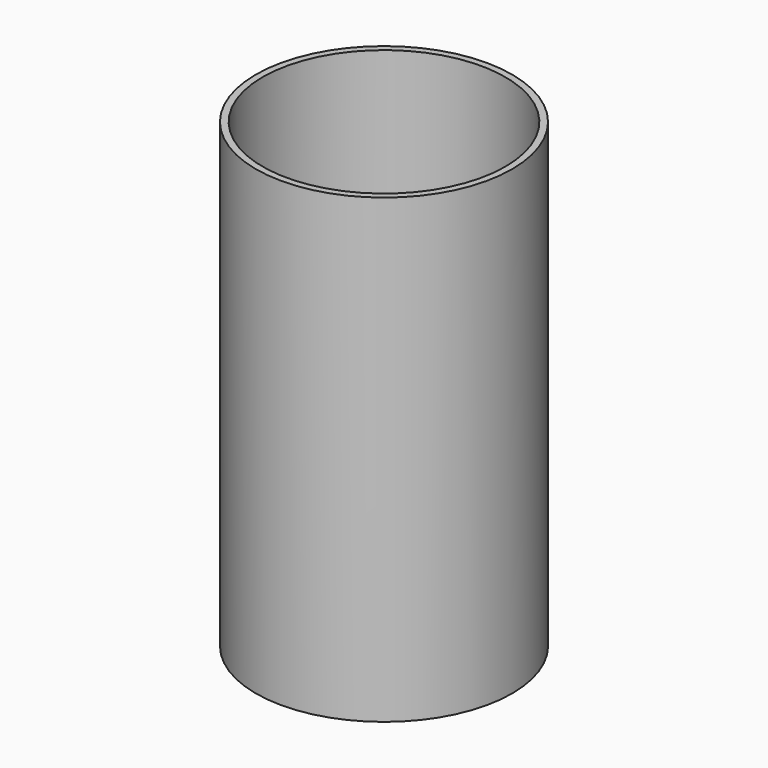
from build123d import *

# Parameters (mm, degrees)
F0_R     = 21.59
F0_R_2   = 20.447
F1_DEPTH = 77.7875


# Not quite as in the source:
# - a length typed as a fraction of an inch, garbled in the dataset ("3 / 203.2 mm" for 3/8 in), is restored


with BuildPart() as f1:
    # F0 (on Top) → F1 (new body)
    with BuildSketch(Plane.XY):
        Circle(F0_R)
        Circle(F0_R_2, mode=Mode.SUBTRACT)
    extrude(amount=F1_DEPTH)


solid = f1.part
